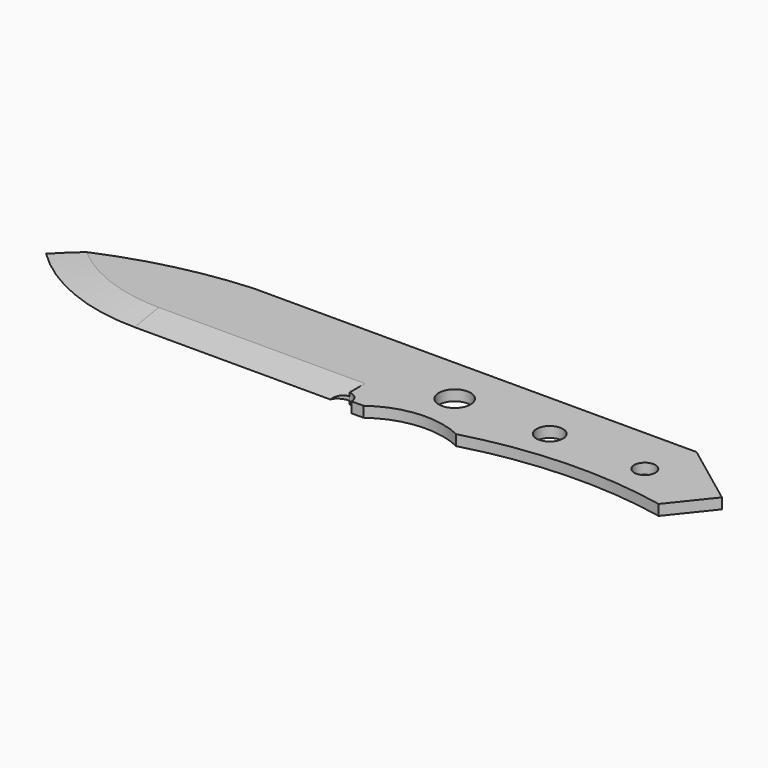
from build123d import *

# Parameters (mm, degrees)
F0_W     = 203.2
F0_H     = 38.1
F1_DEPTH = 3.175
F2_W     = 3.175
F2_H     = 4.445
F3_DEPTH = 25.4


# Not quite as in the source:
# - a feature names something its author has since deleted; it is built from what else it names


with BuildPart() as f1:
    # F0 (on Top) → F1 (new body)
    with BuildSketch(Plane.XY):
        with Locations((101.6, -19.05)):
            Rectangle(F0_W, F0_H)
    extrude(amount=F1_DEPTH)

    # F2 (on face) → F3 (cut)
    with BuildSketch(Plane.XY.offset(3.175)):
        with BuildLine():
            Line((0, -9.525), (0, -14.2875))
            ThreePointArc((0, -14.2875), (24.649723028, -4.4760985439), (50.8, 0))
            Line((50.8, 0), (0, 0))
            Line((0, 0), (0, -9.525))
        make_face()
        with Locations((103.1875, -35.8775)):
            Rectangle(F2_W, F2_H)
        with BuildLine():
            ThreePointArc((104.775, -30.48), (103.8450640303, -32.7250640303), (101.6, -33.655))
            Line((101.6, -33.655), (104.775, -33.655))
            Line((104.775, -33.655), (104.775, -30.48))
        make_face()
        with BuildLine():
            Line((104.775, -30.48), (101.6, -30.48))
            Line((101.6, -30.48), (101.6, -33.655))
            ThreePointArc((101.6, -33.655), (103.8450640303, -32.7250640303), (104.775, -30.48))
        make_face()
        with BuildLine():
            Line((101.6, -27.305), (101.6, -30.48))
            Line((101.6, -30.48), (104.775, -30.48))
            ThreePointArc((104.775, -30.48), (103.8450640303, -28.2349359697), (101.6, -27.305))
        make_face()
        with BuildLine():
            Line((98.4250000029, -30.4801362911), (101.6, -30.48))
            Line((101.6, -30.48), (101.6, -27.305))
            ThreePointArc((101.6, -27.305), (99.3548877841, -28.2349841564), (98.4250000029, -30.4801362911))
        make_face()
        with BuildLine():
            Line((101.6, -33.655), (101.6, -30.48))
            Line((101.6, -30.48), (98.4250000029, -30.4801362911))
            ThreePointArc((98.4250000029, -30.4801362911), (99.3549841564, -32.7251122159), (101.6, -33.655))
        make_face()
        with BuildLine():
            ThreePointArc((108.3690122037, -30.48), (106.4969075417, -31.9824905065), (104.775, -33.655))
            Line((104.775, -33.655), (104.775, -38.1))
            Line((104.775, -38.1), (184.15, -38.1))
            Line((184.15, -38.1), (193.675, -26.19375))
            ThreePointArc((193.675, -26.19375), (163.9135585822, -23.6655567526), (134.3847364187, -28.1581971794))
            ThreePointArc((134.3847364187, -28.1581971794), (121.0555708247, -25.7189035938), (108.3690122037, -30.48))
        make_face()
        with BuildLine():
            Line((101.6, -38.1), (101.6, -33.655))
            ThreePointArc((101.6, -33.655), (99.3549841564, -32.7251122159), (98.4250000029, -30.4801362911))
            Line((98.4250000029, -30.4801362911), (39.6036359929, -30.4826612755))
            ThreePointArc((39.6036359929, -30.4826612755), (18.2099329026, -26.2778753266), (0, -14.2875))
            Line((0, -14.2875), (0, -19.05))
            Line((0, -19.05), (0, -38.1))
            Line((0, -38.1), (101.6, -38.1))
        make_face()
        Polygon((203.2, 0), (184.15, 0), (203.2, -14.2875), align=None)
        Polygon((193.675, -26.19375), (184.15, -38.1), (203.2, -38.1), (203.2, -19.05), (203.2, -14.2875), align=None)
        with BuildLine():
            Line((108.3690122037, -30.48), (104.775, -30.48))
            Line((104.775, -30.48), (104.775, -33.655))
            ThreePointArc((104.775, -33.655), (106.4969075417, -31.9824905065), (108.3690122037, -30.48))
        make_face()
        with BuildLine():
            ThreePointArc((127.6218066335, -14.2875), (122.8593066335, -9.525), (118.0968066335, -14.2875))
            Line((118.0968066335, -14.2875), (127.6218066335, -14.2875))
        make_face()
        with BuildLine():
            Line((127.6218066335, -14.2875), (118.0968066335, -14.2875))
            ThreePointArc((118.0968066335, -14.2875), (122.8593066335, -19.05), (127.6218066335, -14.2875))
        make_face()
        with BuildLine():
            Line((176.8343066335, -14.2875), (183.1843066335, -14.2875))
            ThreePointArc((183.1843066335, -14.2875), (180.0093066335, -11.1125), (176.8343066335, -14.2875))
        make_face()
        with BuildLine():
            ThreePointArc((176.8343066335, -14.2875), (180.0093066335, -17.4625), (183.1843066335, -14.2875))
            Line((183.1843066335, -14.2875), (176.8343066335, -14.2875))
        make_face()
        with BuildLine():
            ThreePointArc((155.4030566335, -14.2875), (151.4343066335, -10.31875), (147.4655566335, -14.2875))
            Line((147.4655566335, -14.2875), (155.4030566335, -14.2875))
        make_face()
        with BuildLine():
            Line((155.4030566335, -14.2875), (147.4655566335, -14.2875))
            ThreePointArc((147.4655566335, -14.2875), (151.4343066335, -18.25625), (155.4030566335, -14.2875))
        make_face()
    extrude(amount=-F3_DEPTH, mode=Mode.SUBTRACT)

    # F8: sweep along a path in F5
    with BuildLine(Plane.XY.offset(1.5875)) as f8_path:
        Line((101.6, -30.48), (39.6036359929, -30.4826612755))
        ThreePointArc((39.6036359929, -30.4826612755), (18.2099329026, -26.2778753266), (0, -14.2875))
    # F7 (on offset) → F8 (sweep, cut)
    with BuildSketch(Plane.YZ.offset(101.6)):
        Polygon((-30.48, 3.1877), (-30.48, 1.5875), (-4.1187478461, 6.2357), (-30.48, 6.2357), align=None)
        Polygon((-30.48, 1.5875), (-30.48, 0), (-30.48, -3.0607), (-4.1187478461, -3.0607), align=None)
    sweep(path=f8_path.line, mode=Mode.SUBTRACT)


solid = f1.part
